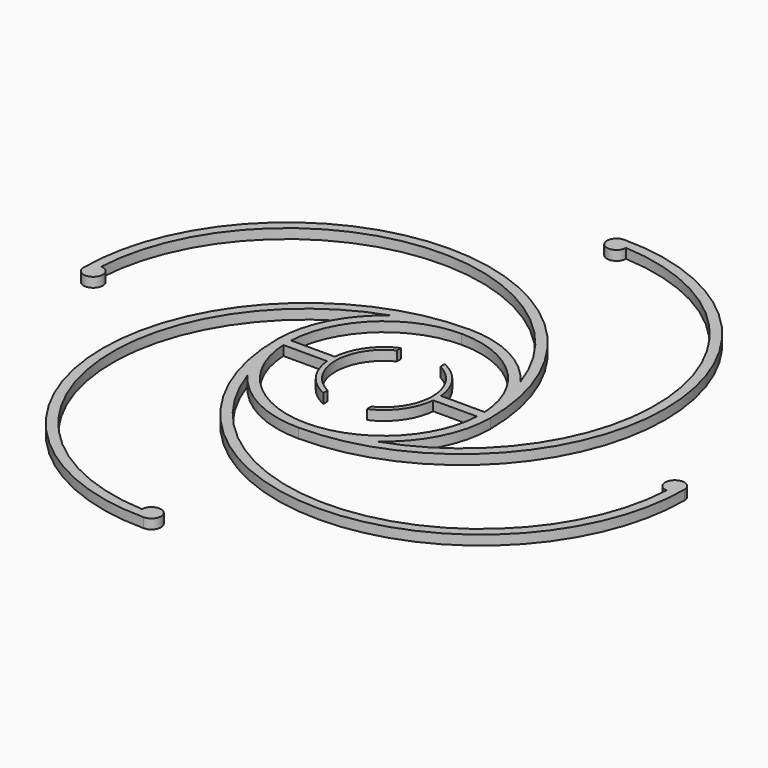
from build123d import *

# Parameters (mm, degrees)
F1_DEPTH   = 1
F1_FACE_W  = 1
F1_FACE_H  = 1
F1_FACE1_W = 1
F1_FACE1_H = 1
F1_FACE2_W = 1
F1_FACE2_H = 1
F1_FACE3_W = 1
F1_FACE3_H = 1


# Not quite as in the source:
# - a feature names something its author has since deleted; it is built from what else it names


with BuildPart() as f1:
    # F0 (on Top) → F1 (new body)
    with BuildSketch(Plane.XY):
        with BuildLine():
            ThreePointArc((8.95, 6.3951153234), (9.735754356, 3.2403703492), (10, 0))
            ThreePointArc((10, 0), (9.9968982101, -0.2490505519), (9.9875947645, -0.4979466032))
            ThreePointArc((9.9875947645, -0.4979466032), (6.8927691811, -7.2449798493), (0, -10))
            ThreePointArc((0, -10), (3.2403703492, -9.735754356), (6.3951153234, -8.95))
            ThreePointArc((6.3951153234, -8.95), (9.7812644519, -5.0325804237), (11, 0))
            ThreePointArc((11, 0), (10.474970167, 3.3578266781), (8.95, 6.3951153234))
        make_face()
        with BuildLine():
            ThreePointArc((9.9875947645, 0.4979466032), (9.9968982101, 0.2490505519), (10, 0))
            ThreePointArc((10, 0), (9.735754356, 3.2403703492), (8.95, 6.3951153234))
            ThreePointArc((8.95, 6.3951153234), (5.0325804237, 9.7812644519), (0, 11))
            ThreePointArc((0, 11), (-3.3578266781, 10.474970167), (-6.3951153234, 8.95))
            ThreePointArc((-6.3951153234, 8.95), (-3.2403703492, 9.735754356), (0, 10))
            ThreePointArc((0, 10), (6.8927691811, 7.2449798493), (9.9875947645, 0.4979466032))
        make_face()
        with BuildLine():
            ThreePointArc((-30, 0), (-13.2403703492, 19.735754356), (8.95, 6.3951153234))
            ThreePointArc((8.95, 6.3951153234), (10.474970167, 3.3578266781), (11, 0))
            ThreePointArc((11, 0), (-10, 21), (-31, 0))
            Line((-31, 0), (-30, 0))
        make_face()
        with BuildLine():
            ThreePointArc((-9.9875233888, 0.4993761694), (-6.8922506595, 7.2454731279), (0, 10))
            ThreePointArc((0, 10), (-3.2403703492, 9.735754356), (-6.3951153234, 8.95))
            ThreePointArc((-6.3951153234, 8.95), (-9.7812644519, 5.0325804237), (-11, 0))
            ThreePointArc((-11, 0), (-10.474970167, -3.3578266781), (-8.95, -6.3951153234))
            ThreePointArc((-8.95, -6.3951153234), (-9.735754356, -3.2403703492), (-10, 0))
            ThreePointArc((-10, 0), (-9.9968803606, 0.2497660027), (-9.9875233888, 0.4993761694))
        make_face()
        with BuildLine():
            ThreePointArc((6.3951153234, -8.95), (3.2403703492, -9.735754356), (0, -10))
            ThreePointArc((0, -10), (-6.8922506595, -7.2454731279), (-9.9875233888, -0.4993761694))
            ThreePointArc((-9.9875233888, -0.4993761694), (-9.9968803606, -0.2497660027), (-10, 0))
            ThreePointArc((-10, 0), (-9.735754356, -3.2403703492), (-8.95, -6.3951153234))
            ThreePointArc((-8.95, -6.3951153234), (-5.0325804237, -9.7812644519), (0, -11))
            ThreePointArc((0, -11), (3.3578266781, -10.474970167), (6.3951153234, -8.95))
        make_face()
        with BuildLine():
            ThreePointArc((-6.3951153234, 8.95), (-3.3578266781, 10.474970167), (0, 11))
            ThreePointArc((0, 11), (-21, -10), (0, -31))
            Line((0, -31), (0, -30))
            ThreePointArc((0, -30), (-19.735754356, -13.2403703492), (-6.3951153234, 8.95))
        make_face()
        with BuildLine():
            ThreePointArc((0, 30), (19.735754356, 13.2403703492), (6.3951153234, -8.95))
            ThreePointArc((6.3951153234, -8.95), (3.3578266781, -10.474970167), (0, -11))
            ThreePointArc((0, -11), (21, 10), (0, 31))
            Line((0, 31), (0, 30))
        make_face()
        with BuildLine():
            ThreePointArc((-8.95, -6.3951153234), (-10.474970167, -3.3578266781), (-11, 0))
            ThreePointArc((-11, 0), (10, -21), (31, 0))
            Line((31, 0), (30, 0))
            ThreePointArc((30, 0), (13.2403703492, -19.735754356), (-8.95, -6.3951153234))
        make_face()
        with BuildLine():
            ThreePointArc((5.5, 0), (5.4943502571, 0.2492293164), (5.4774126356, 0.4979466032))
            ThreePointArc((5.4774126356, 0.4979466032), (4.4763336759, 3.1956903514), (2.25, 5.018714975))
            Line((2.25, 5.018714975), (2.25, 4.4651427749))
            ThreePointArc((2.25, 4.4651427749), (4.2573465915, 2.6220221204), (5, 0))
            ThreePointArc((5, 0), (4.2573465915, -2.6220221204), (2.25, -4.4651427749))
            Line((2.25, -4.4651427749), (2.25, -5.018714975))
            ThreePointArc((2.25, -5.018714975), (4.4763336759, -3.1956903514), (5.4774126356, -0.4979466032))
            ThreePointArc((5.4774126356, -0.4979466032), (5.4943502571, -0.2492293164), (5.5, 0))
        make_face()
        with BuildLine():
            ThreePointArc((9.9875947645, -0.4979466032), (9.9968982101, -0.2490505519), (10, 0))
            ThreePointArc((10, 0), (9.9968982101, 0.2490505519), (9.9875947645, 0.4979466032))
            Line((9.9875947645, 0.4979466032), (5.4774126356, 0.4979466032))
            ThreePointArc((5.4774126356, 0.4979466032), (5.4943502571, 0.2492293164), (5.5, 0))
            ThreePointArc((5.5, 0), (5.4943502571, -0.2492293164), (5.4774126356, -0.4979466032))
            Line((5.4774126356, -0.4979466032), (9.9875947645, -0.4979466032))
        make_face()
        with BuildLine():
            ThreePointArc((-2.25, 5.018714975), (-4.4761862714, 3.1958968168), (-5.4773666772, 0.4984518873))
            ThreePointArc((-5.4773666772, 0.4984518873), (-5.5, 0), (-5.4773666772, -0.4984518873))
            ThreePointArc((-5.4773666772, -0.4984518873), (-4.4761862714, -3.1958968168), (-2.25, -5.018714975))
            Line((-2.25, -5.018714975), (-2.25, -4.4651427749))
            ThreePointArc((-2.25, -4.4651427749), (-5, 0), (-2.25, 4.4651427749))
            Line((-2.25, 4.4651427749), (-2.25, 5.018714975))
        make_face()
        with BuildLine():
            Line((-5.4773666772, 0.4984518873), (-9.9875233888, 0.4993761694))
            ThreePointArc((-9.9875233888, 0.4993761694), (-9.9968803606, 0.2497660027), (-10, 0))
            ThreePointArc((-10, 0), (-9.9968803606, -0.2497660027), (-9.9875233888, -0.4993761694))
            Line((-9.9875233888, -0.4993761694), (-5.4773666772, -0.4984518873))
            ThreePointArc((-5.4773666772, -0.4984518873), (-5.5, 0), (-5.4773666772, 0.4984518873))
        make_face()
    extrude(amount=F1_DEPTH)

    # F1_face (on face) → F2 (revolve)
    with BuildSketch(Plane(origin=(-30.5, 0, 0.5), x_dir=(1, 0, 0), z_dir=(0, -1, 0))):
        Rectangle(F1_FACE_W, F1_FACE_H)
    revolve(axis=Axis((-30, 0, 0.5), (0, 0, -1)))

    # F1_face1 (on face) → F3 (revolve)
    with BuildSketch(Plane(origin=(0, -30.5, 0.5), x_dir=(0, 1, 0), z_dir=(1, 0, 0))):
        Rectangle(F1_FACE1_W, F1_FACE1_H)
    revolve(axis=Axis((0, -30, 0.5), (0, 0, -1)))

    # F1_face2 (on face) → F4 (revolve)
    with BuildSketch(Plane(origin=(30.5, 0, 0.5), x_dir=(-1, 0, 0), z_dir=(0, 1, 0))):
        Rectangle(F1_FACE2_W, F1_FACE2_H)
    revolve(axis=Axis((30, 0, 0.5), (0, 0, -1)))

    # F1_face3 (on face) → F5 (revolve)
    with BuildSketch(Plane(origin=(0, 30.5, 0.5), x_dir=(0, -1, 0), z_dir=(-1, 0, 0))):
        Rectangle(F1_FACE3_W, F1_FACE3_H)
    revolve(axis=Axis((0, 30, 0.5), (0, 0, -1)))


solid = f1.part
